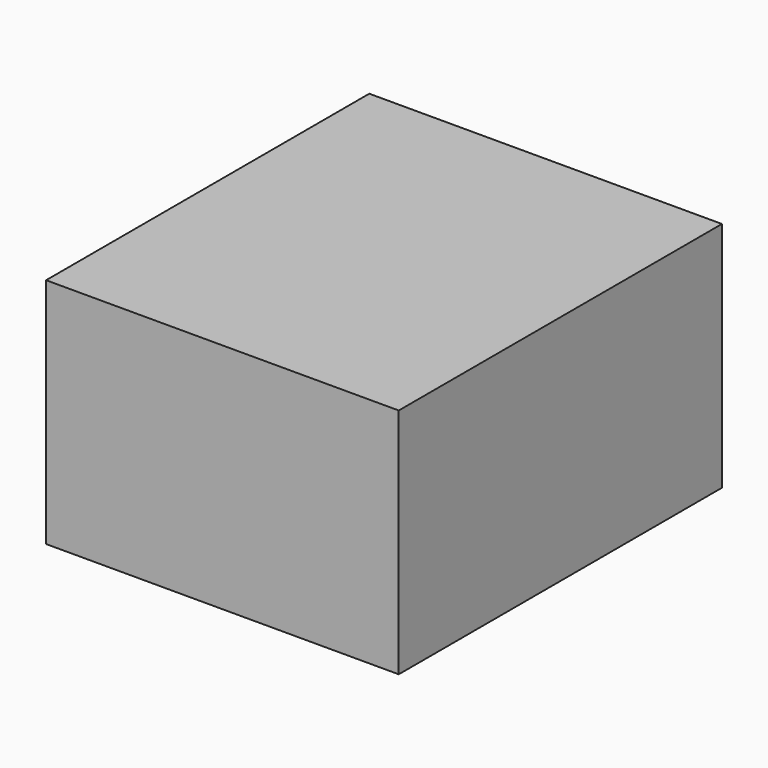
from build123d import *

# Parameters (mm, degrees)
F1_DEPTH       = 25.4
F2_START       = 6.35
F2_DEPTH       = 12.7
F4_R           = 3.175
F5_DEPTH       = 12.7
F9_ANGLE       = 180
F12_START      = 15.875
F12_DEPTH      = 6.35
F13_DEPTH      = 8.89
F13_DEPTH_BACK = 3.175
F15_W          = 221.7474803329
F15_H          = 146.0437215865
F16_DEPTH      = 254


# Not quite as in the source:
# - the program builds the solid bodies; features that only make, move or delete a surface that nothing else refers to are left out


with BuildPart() as f1:
    # F0 (on Front) → F1 (new body)
    with BuildSketch(Plane.XZ):
        with BuildLine():
            ThreePointArc((-19.05, 0), (-23.5359997431, 12.2797555561), (-34.8812227315, 18.7761011101))
            add(Edge.make_bspline(
                [(-34.8812227315, 18.7761011101), (-35.9539739891, 18.8673096465), (-37.0269869945, 18.9586548233), (-38.1, 19.05)],
                knots=[0.9852412325, 0.9852412325, 0.9852412325, 0.9852412325, 1, 1, 1, 1], degree=3))
            ThreePointArc((-38.1, 19.05), (-51.5703841816, 13.4703841816), (-57.15, 0))
            ThreePointArc((-57.15, 0), (-51.5703841816, -13.4703841816), (-38.1, -19.05))
            add(Edge.make_bspline(
                [(-34.8812227315, -18.7761011101), (-35.9539739891, -18.8673096465), (-37.0269869945, -18.9586548233), (-38.1, -19.05)],
                knots=[0.9852412325, 0.9852412325, 0.9852412325, 0.9852412325, 1, 1, 1, 1], degree=3))
            ThreePointArc((-34.8812227315, -18.7761011101), (-23.5359997431, -12.2797555561), (-19.05, 0))
        make_face()
        with BuildLine():
            ThreePointArc((-25.4, 0), (-38.1, -12.7), (-50.8, 0))
            ThreePointArc((-50.8, 0), (-38.1, 12.7), (-25.4, 0))
        make_face(mode=Mode.SUBTRACT)
    extrude(amount=F1_DEPTH)


with BuildPart() as f1b:
    # F0 (on Front) → F1, piece 2 (new body)
    with BuildSketch(Plane.XZ):
        with BuildLine():
            ThreePointArc((101.6, 0), (109.0394877579, 17.9605122421), (127, 25.4))
            Line((127, 25.4), (127, 31.75))
            ThreePointArc((127, 31.75), (104.5493596973, 22.4506403027), (95.25, 0))
            ThreePointArc((95.25, 0), (104.5493596973, -22.4506403027), (127, -31.75))
            Line((127, -31.75), (127, -25.4))
            ThreePointArc((127, -25.4), (109.0394877579, -17.9605122421), (101.6, 0))
        make_face()
    extrude(amount=F1_DEPTH)


with BuildPart() as f2:
    # F0 (on Front) → F2 (new body)
    with BuildSketch(Plane.XZ.offset(F2_START)):
        with BuildLine():
            ThreePointArc((95.25, 0), (104.5493596973, 22.4506403027), (127, 31.75))
            Line((127, 31.75), (127, 38.1))
            Line((127, 38.1), (114.3, 38.1))
            Line((114.3, 38.1), (107.95, 38.1))
            add(Edge.make_bspline(
                [(107.95, 38.1), (101.5454845618, 30.6734948539), (82.9350516774, 9.0933336503), (12.0871454681, 14.7827092653), (-34.8812227315, 18.7761011101)],
                knots=[0, 0, 0, 0, 0.3390567389, 0.9852412325, 0.9852412325, 0.9852412325, 0.9852412325], degree=3))
            ThreePointArc((-34.8812227315, 18.7761011101), (-23.5359997431, 12.2797555561), (-19.05, 0))
            ThreePointArc((-19.05, 0), (-23.5359997431, -12.2797555561), (-34.8812227315, -18.7761011101))
            add(Edge.make_bspline(
                [(107.95, -38.1), (101.5454845618, -30.6734948539), (82.9350516774, -9.0933336503), (12.0871454681, -14.7827092653), (-34.8812227315, -18.7761011101)],
                knots=[0, 0, 0, 0, 0.3390567389, 0.9852412325, 0.9852412325, 0.9852412325, 0.9852412325], degree=3))
            Line((107.95, -38.1), (114.3, -38.1))
            Line((114.3, -38.1), (127, -38.1))
            Line((127, -38.1), (127, -31.75))
            ThreePointArc((127, -31.75), (104.5493596973, -22.4506403027), (95.25, 0))
        make_face()
    extrude(amount=F2_DEPTH)

    # F11 (on Front) → F12 (cut)
    with BuildSketch(Plane.XZ.offset(F12_START)):
        with BuildLine():
            ThreePointArc((76.9020138437, -5.1012635231), (70.5520138437, 1.2487364769), (76.9020138437, 7.5987364769))
            Line((76.9020138437, 7.5987364769), (76.9020138437, 7.637041232))
            Line((76.9020138437, 7.637041232), (0.7020138437, 7.637041232))
            ThreePointArc((0.7020138437, 7.637041232), (5.2192274563, 5.7659500895), (7.0903185988, 1.2487364769))
            ThreePointArc((7.0903185988, 1.2487364769), (5.4597880273, -3.014363623), (1.4005391789, -5.1012635231))
            Line((1.4005391789, -5.1012635231), (76.9020138437, -5.1012635231))
        make_face()
        with BuildLine():
            Line((0.7020138437, -5.1012635231), (1.4005391789, -5.1012635231))
            ThreePointArc((1.4005391789, -5.1012635231), (5.4597880273, -3.014363623), (7.0903185988, 1.2487364769))
            ThreePointArc((7.0903185988, 1.2487364769), (5.2192274563, 5.7659500895), (0.7020138437, 7.637041232))
            Line((0.7020138437, 7.637041232), (0.7020138437, -5.1012635231))
        make_face()
        with BuildLine():
            ThreePointArc((0.7020138437, 7.637041232), (-5.6767075344, 0.8989490778), (1.4005391789, -5.1012635231))
            Line((1.4005391789, -5.1012635231), (0.7020138437, -5.1012635231))
            Line((0.7020138437, -5.1012635231), (0.7020138437, 7.637041232))
        make_face()
        with BuildLine():
            Line((76.9020138437, -5.1012635231), (76.9020138437, 7.5987364769))
            ThreePointArc((76.9020138437, 7.5987364769), (70.5520138437, 1.2487364769), (76.9020138437, -5.1012635231))
        make_face()
        with BuildLine():
            ThreePointArc((76.9020138437, -5.1012635231), (81.3921419042, -3.2413915836), (83.2520138437, 1.2487364769))
            ThreePointArc((83.2520138437, 1.2487364769), (81.3921419042, 5.7388645374), (76.9020138437, 7.5987364769))
            Line((76.9020138437, 7.5987364769), (76.9020138437, -5.1012635231))
        make_face()
    extrude(amount=F12_DEPTH, mode=Mode.SUBTRACT)

    # F11 (on Front) → F13 (cut, two sides)
    with BuildSketch(Plane.XZ) as f13_sk:
        with BuildLine():
            ThreePointArc((76.9020138437, -5.1012635231), (70.5520138437, 1.2487364769), (76.9020138437, 7.5987364769))
            Line((76.9020138437, 7.5987364769), (76.9020138437, 7.637041232))
            Line((76.9020138437, 7.637041232), (0.7020138437, 7.637041232))
            ThreePointArc((0.7020138437, 7.637041232), (5.2192274563, 5.7659500895), (7.0903185988, 1.2487364769))
            ThreePointArc((7.0903185988, 1.2487364769), (5.4597880273, -3.014363623), (1.4005391789, -5.1012635231))
            Line((1.4005391789, -5.1012635231), (76.9020138437, -5.1012635231))
        make_face()
        with BuildLine():
            Line((0.7020138437, -5.1012635231), (1.4005391789, -5.1012635231))
            ThreePointArc((1.4005391789, -5.1012635231), (5.4597880273, -3.014363623), (7.0903185988, 1.2487364769))
            ThreePointArc((7.0903185988, 1.2487364769), (5.2192274563, 5.7659500895), (0.7020138437, 7.637041232))
            Line((0.7020138437, 7.637041232), (0.7020138437, -5.1012635231))
        make_face()
        with BuildLine():
            ThreePointArc((0.7020138437, 7.637041232), (-5.6767075344, 0.8989490778), (1.4005391789, -5.1012635231))
            Line((1.4005391789, -5.1012635231), (0.7020138437, -5.1012635231))
            Line((0.7020138437, -5.1012635231), (0.7020138437, 7.637041232))
        make_face()
        with BuildLine():
            ThreePointArc((76.9020138437, -5.1012635231), (81.3921419042, -3.2413915836), (83.2520138437, 1.2487364769))
            ThreePointArc((83.2520138437, 1.2487364769), (81.3921419042, 5.7388645374), (76.9020138437, 7.5987364769))
            Line((76.9020138437, 7.5987364769), (76.9020138437, -5.1012635231))
        make_face()
        with BuildLine():
            Line((76.9020138437, -5.1012635231), (76.9020138437, 7.5987364769))
            ThreePointArc((76.9020138437, 7.5987364769), (70.5520138437, 1.2487364769), (76.9020138437, -5.1012635231))
        make_face()
    extrude(amount=F13_DEPTH, mode=Mode.SUBTRACT)
    extrude(f13_sk.sketch, amount=-F13_DEPTH_BACK, mode=Mode.SUBTRACT)


with BuildPart() as f5:
    # F4 (on Right) → F5 (new body)
    with BuildSketch(Plane.YZ):
        with BuildLine():
            Line((-6.318667513, 31.7657962441), (-6.3902429704, 38.1010105191))
            ThreePointArc((-6.3902429704, 38.1010105191), (-12.701443823, 45.1269305241), (-19.018667513, 38.106425345))
            Line((-19.018667513, 38.106425345), (-19.018667513, 31.7657962441))
            Line((-19.018667513, 31.7657962441), (-6.318667513, 31.7657962441))
        make_face()
        with Locations((-12.7041665808, 38.7769311078)):
            Circle(F4_R, mode=Mode.SUBTRACT)
    extrude(amount=F5_DEPTH)


with BuildPart() as f5_1:
    # F6: moved
    add(f5.part.moved(Location((107.95, 0, 3.175))))


with BuildPart() as f7_1:
    # F7: copy of F5
    add(f5_1.part)


with BuildPart() as f7_1_1:
    # F8: moved
    add(f7_1.part.moved(Location((26.162, 0, -77.216))))


with BuildPart() as f7_1_2:
    # F9: moved
    add(f7_1_1.part.rotate(Axis((140.462, -19.018667513, -35.934574655), (1, 0, 0)), F9_ANGLE))


with BuildPart() as f7_1_3:
    # F10: moved
    add(f7_1_2.part.moved(Location((-26.1747, 12.7, -6.35))))


with BuildPart() as f5_2:
    # F14: moved
    add(f5_1.part.moved(Location((6.35, 0, 0))))


with BuildPart() as f7_1_4:
    # F14: moved
    add(f7_1_3.part.moved(Location((6.35, 0, 0))))


with BuildPart() as f16:
    # F15 (on Front) → F16 (new body)
    with BuildSketch(Plane.XZ):
        with Locations((29.3813087046, -11.6117652506)):
            Rectangle(F15_W, F15_H)
    extrude(amount=F16_DEPTH)


solid = Compound([f1.part, f1b.part, f2.part, f5_2.part, f7_1_4.part, f16.part])
